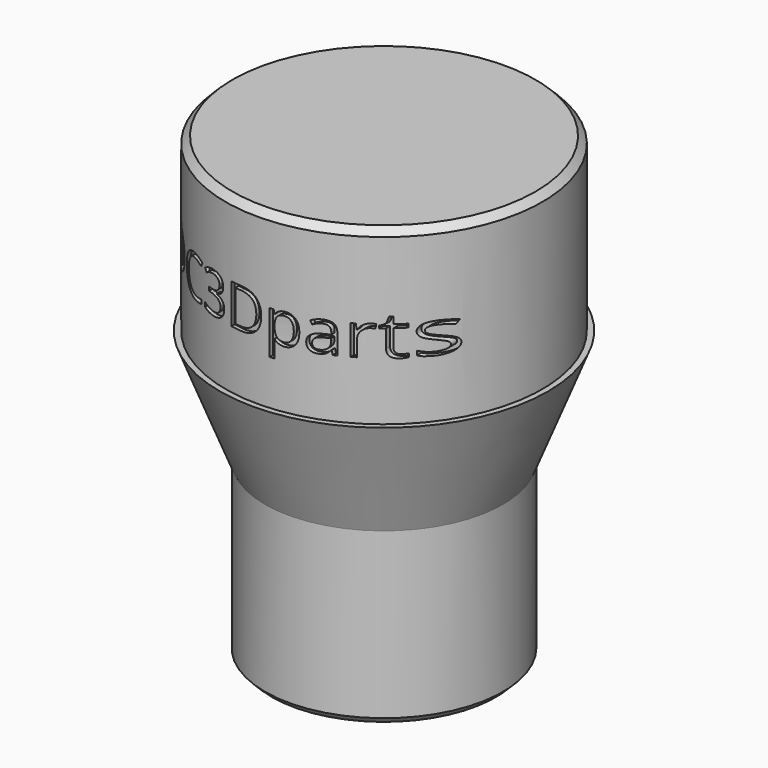
from build123d import *

# Parameters (mm, degrees)
F2_SIZE      = 1.2
F4_TEXT_SIZE = 9.7222222222
F5_DEPTH     = 40
F6_W         = 27
F6_H         = 32.225641878


# Not quite as in the source:
# - Text() gives the source's letters only with a copy of the font that has no kerning and outlines rounded to 1/6400 em; it was checked with that copy


with BuildPart() as f1:
    # F0 (on Front) → F1 (revolve)
    with BuildSketch(Plane.XZ):
        Polygon((0, 73.2666279856), (-27.685, 73.2666279856), (-27.685, 43.2666279856), (-28.7, 43.2666279856), (-20.8, 23.2666279856), (-20.8, -6.7333720144), (0, -6.7333720144), align=None)
    revolve(axis=Axis((0, 0, -2.5966958965), (0, 0, -1)))

    # F2
    f2_edges = [f1.edges().sort_by_distance(p)[0] for p in [
        (27.685, 0, 73.266628),
        (20.8, 0, -6.733372),
    ]]
    chamfer(f2_edges, length=F2_SIZE)


with BuildPart() as f5:
    # F4 (on offset) → F5 (new body, through all)
    with BuildSketch(Plane.XZ.offset(40)):
        with Locations((-24.5914840117, 53.4490973013)):
            Text('DC3Dparts', F4_TEXT_SIZE, font='Open Sans', text_align=(TextAlign.LEFT, TextAlign.BOTTOM))
    extrude(amount=-F5_DEPTH)


with BuildPart() as f7:
    # F6 (on Front) → F7 (revolve)
    with BuildSketch(Plane.XZ):
        with Locations((-13.5, 63.0638580157)):
            Rectangle(F6_W, F6_H)
    revolve(axis=Axis((0, 0, 63.0638580157), (0, 0, 1)))


with BuildPart() as f5_1:
    add(f5.part)

    # F8: cut F7
    add(f7.part, mode=Mode.SUBTRACT)


with BuildPart() as f1_1:
    add(f1.part)

    # F9: cut F5
    add(f5_1.part, mode=Mode.SUBTRACT)


solid = f1_1.part
